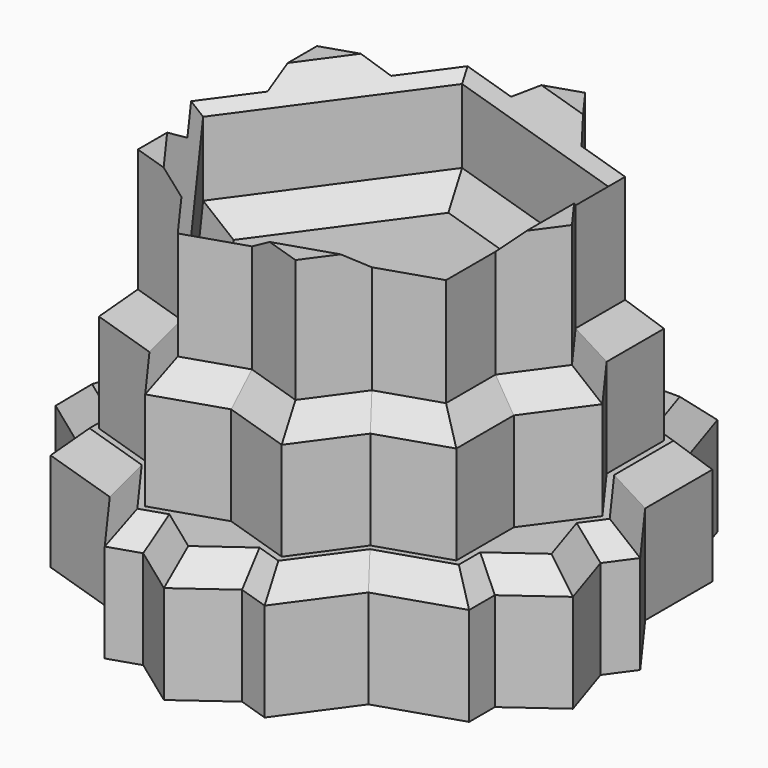
from build123d import *

# Parameters (mm, degrees)
F1_DEPTH      = 25.4
F2_SIZE       = 5.08
F4_DEPTH      = 25.4
F5_SIZE       = 5.08
F7_DEPTH      = 25.4
F8_SIZE       = 5.08
F9_T4_DEPTH   = 69.3683527658
F9_T10_DEPTH  = 69.3683527658
F9_T16_DEPTH  = 69.3683527658
F9_T22_DEPTH  = 69.3683527658
F9_T28_DEPTH  = 69.3683527658
F9_T35_DEPTH  = 69.3683527658
F9_T41_DEPTH  = 69.3683527658
F9_T50_DEPTH  = 69.3683527658
F9_T56_DEPTH  = 69.3683527658
F9_T65_DEPTH  = 69.3683527658
F9_T71_DEPTH  = 69.3683527658
F9_T80_DEPTH  = 69.3683527658
F9_T86_DEPTH  = 69.3683527658
F9_T95_DEPTH  = 69.3683527658
F9_T101_DEPTH = 69.3683527658


# Not quite as in the source:
# - a fillet or chamfer that OpenCascade refuses, or shapes differently, is made with other operations: its cross-section is extruded or revolved along the edge and cut away or added


with BuildPart() as f1:
    # F0 (on Top) → F1 (new body)
    with BuildSketch(Plane.XY):
        Polygon((43.1581027806, 14.0229176455), (43.1581027806, 31.3561970981), (36.8614204445, 33.40211321), align=None)
        Polygon((49.4547851167, -5.3562779191), (43.1581027806, 14.0229176455), (43.1581027806, -14.0229176455), align=None)
        Polygon((43.1581027806, -14.0229176455), (43.1581027806, 14.0229176455), (26.6731744084, 36.7124750172), (0, 45.3791147436), (-26.6731744084, 36.7124750172), (-43.1581027806, 14.0229176455), (-43.1581027806, -14.0229176455), (-26.6731744084, -36.7124750172), (0, -45.3791147436), (26.6731744084, -36.7124750172), align=None)
        Polygon((26.6731744084, 36.7124750172), (43.1581027806, 14.0229176455), (36.8614204445, 33.40211321), align=None)
        Polygon((53.3463488167, 0), (43.1581027806, 14.0229176455), (49.4547851167, -5.3562779191), align=None)
        Polygon((26.6731744084, 36.7124750172), (36.8614204445, 33.40211321), (32.9698567444, 45.3791147436), (20.3764920723, 45.3791147436), align=None)
        Polygon((49.4547851167, -5.3562779191), (43.1581027806, -14.0229176455), (43.1581027806, -24.7354734837), (53.3463488167, -17.3332794527), align=None)
        Polygon((43.1581027806, -24.7354734837), (43.1581027806, -14.0229176455), (26.6731744084, -36.7124750172), align=None)
        Polygon((0, 45.3791147436), (26.6731744084, 36.7124750172), (20.3764920723, 45.3791147436), align=None)
        Polygon((43.1581027806, -31.3561970981), (43.1581027806, -24.7354734837), (26.6731744084, -36.7124750172), align=None)
        Polygon((10.1882460361, -48.6894765508), (26.6731744084, -36.7124750172), (0, -45.3791147436), align=None)
        Polygon((16.4849283722, -50.7353926627), (26.6731744084, -36.7124750172), (10.1882460361, -48.6894765508), align=None)
        Polygon((-20.3764920723, 45.3791147436), (0, 45.3791147436), (-16.4849283722, 50.7353926627), align=None)
        Polygon((-26.6731744084, 36.7124750172), (0, 45.3791147436), (-20.3764920723, 45.3791147436), align=None)
        Polygon((16.4849283722, 50.7353926627), (0, 45.3791147436), (20.3764920723, 45.3791147436), align=None)
        Polygon((10.1882460361, -48.6894765508), (0, -45.3791147436), (-10.1882460361, -48.6894765508), (0, -56.0916705818), align=None)
        Polygon((-10.1882460361, -48.6894765508), (0, -45.3791147436), (-26.6731744084, -36.7124750172), align=None)
        Polygon((-36.8614204445, 33.40211321), (-26.6731744084, 36.7124750172), (-20.3764920723, 45.3791147436), (-32.9698567444, 45.3791147436), align=None)
        Polygon((-43.1581027806, 14.0229176455), (-26.6731744084, 36.7124750172), (-36.8614204445, 33.40211321), align=None)
        Polygon((-16.4849283722, -50.7353926627), (-10.1882460361, -48.6894765508), (-26.6731744084, -36.7124750172), align=None)
        Polygon((-43.1581027806, -24.7354734837), (-26.6731744084, -36.7124750172), (-43.1581027806, -14.0229176455), align=None)
        Polygon((-43.1581027806, -31.3561970981), (-26.6731744084, -36.7124750172), (-43.1581027806, -24.7354734837), align=None)
        Polygon((-49.4547851167, -5.3562779191), (-43.1581027806, 14.0229176455), (-53.3463488167, 0), align=None)
        Polygon((-43.1581027806, -14.0229176455), (-43.1581027806, 14.0229176455), (-49.4547851167, -5.3562779191), align=None)
        Polygon((-43.1581027806, 31.3561970981), (-43.1581027806, 14.0229176455), (-36.8614204445, 33.40211321), align=None)
        Polygon((-43.1581027806, -24.7354734837), (-43.1581027806, -14.0229176455), (-49.4547851167, -5.3562779191), (-53.3463488167, -17.3332794527), align=None)
    extrude(amount=F1_DEPTH)

    # F2
    f2_edges = [f1.edges().sort_by_distance(p)[0] for p in [
        (43.158103, 22.689557, 25.4),
        (40.009762, 32.379155, 25.4),
        (34.915639, 39.390614, 25.4),
        (26.673174, 45.379115, 25.4),
        (18.43071, 48.057254, 25.4),
        (8.242464, 48.057254, 25.4),
        (-8.242464, 48.057254, 25.4),
        (-18.43071, 48.057254, 25.4),
        (-26.673174, 45.379115, 25.4),
        (-34.915639, 39.390614, 25.4),
        (-40.009762, 32.379155, 25.4),
        (-43.158103, 22.689557, 25.4),
        (-48.252226, 7.011459, 25.4),
        (-51.400567, -2.678139, 25.4),
        (-51.400567, -11.344779, 25.4),
        (-48.252226, -21.034376, 25.4),
        (-43.158103, -28.045835, 25.4),
        (-34.915639, -34.034336, 25.4),
        (-21.579051, -43.723934, 25.4),
        (-13.336587, -49.712435, 25.4),
        (-5.094123, -52.390574, 25.4),
        (5.094123, -52.390574, 25.4),
        (13.336587, -49.712435, 25.4),
        (21.579051, -43.723934, 25.4),
        (34.915639, -34.034336, 25.4),
        (43.158103, -28.045835, 25.4),
        (48.252226, -21.034376, 25.4),
        (51.400567, -11.344779, 25.4),
        (51.400567, -2.678139, 25.4),
        (48.252226, 7.011459, 25.4),
    ]]
    chamfer(f2_edges, length=F2_SIZE)

    # F3 (on face) → F4 (join)
    with BuildSketch(Plane.XY.offset(25.4)):
        Polygon((36.8518978357, 11.9739074504), (36.8518978357, 26.7744710154), (22.7757254124, 31.3480966833), align=None)
        Polygon((45.5514508248, 0), (36.8518978357, 11.9739074504), (36.8518978357, -11.9739074504), align=None)
        Polygon((36.8518978357, -11.9739074504), (36.8518978357, 11.9739074504), (22.7757254124, 31.3480966833), (0, 38.7483784658), (-22.7757254124, 31.3480966833), (-36.8518978357, 11.9739074504), (-36.8518978357, -11.9739074504), (-22.7757254124, -31.3480966833), (0, -38.7483784658), (22.7757254124, -31.3480966833), align=None)
        Polygon((0, 38.7483784658), (22.7757254124, 31.3480966833), (14.0761724233, 43.3220041337), align=None)
        Polygon((36.8518978357, -26.7744710154), (36.8518978357, -11.9739074504), (22.7757254124, -31.3480966833), align=None)
        Polygon((-22.7757254124, 31.3480966833), (0, 38.7483784658), (-14.0761724233, 43.3220041337), align=None)
        Polygon((14.0761724233, -43.3220041337), (22.7757254124, -31.3480966833), (0, -38.7483784658), align=None)
        Polygon((-36.8518978357, 11.9739074504), (-22.7757254124, 31.3480966833), (-36.8518978357, 26.7744710154), align=None)
        Polygon((-14.0761724233, -43.3220041337), (0, -38.7483784658), (-22.7757254124, -31.3480966833), align=None)
        Polygon((-36.8518978357, -11.9739074504), (-36.8518978357, 11.9739074504), (-45.5514508248, 0), align=None)
        Polygon((-36.8518978357, -26.7744710154), (-22.7757254124, -31.3480966833), (-36.8518978357, -11.9739074504), align=None)
    extrude(amount=F4_DEPTH)

    # F5
    f5_edges = [f1.edges().sort_by_distance(p)[0] for p in [
        (36.851898, 19.374189, 50.8),
        (29.813812, 29.061284, 50.8),
        (18.425949, 37.33505, 50.8),
        (7.038086, 41.035191, 50.8),
        (-7.038086, 41.035191, 50.8),
        (-18.425949, 37.33505, 50.8),
        (-29.813812, 29.061284, 50.8),
        (-36.851898, 19.374189, 50.8),
        (-41.201674, 5.986954, 50.8),
        (-41.201674, -5.986954, 50.8),
        (-36.851898, -19.374189, 50.8),
        (-29.813812, -29.061284, 50.8),
        (-18.425949, -37.33505, 50.8),
        (-7.038086, -41.035191, 50.8),
        (7.038086, -41.035191, 50.8),
        (18.425949, -37.33505, 50.8),
        (29.813812, -29.061284, 50.8),
        (36.851898, -19.374189, 50.8),
        (41.201674, -5.986954, 50.8),
        (41.201674, 5.986954, 50.8),
    ]]
    chamfer(f5_edges, length=F5_SIZE)

    # F6 (on face) → F7 (join)
    with BuildSketch(Plane.XY.offset(50.8)):
        Polygon((39.2722254991, 0), (31.7718978357, 10.3233153935), (31.7718978357, 23.0836349731), (19.6361127496, 27.0267905768), (12.1357850862, 37.3501059704), (0, 33.4069503666), (-12.1357850862, 37.3501059704), (-19.6361127496, 27.0267905768), (-31.7718978357, 23.0836349731), (-31.7718978357, 10.3233153935), (-39.2722254991, 0), (-31.7718978357, -10.3233153935), (-31.7718978357, -23.0836349731), (-19.6361127496, -27.0267905768), (-12.1357850862, -37.3501059704), (0, -33.4069503666), (12.1357850862, -37.3501059704), (19.6361127496, -27.0267905768), (31.7718978357, -23.0836349731), (31.7718978357, -10.3233153935), align=None)
        Polygon((-11.3663207357, 34.9819382066), (29.7574140131, 21.620026804), (29.7574140131, -21.620026804), (-11.3663207357, -34.9819382066), (-36.7821865549, 0), align=None, mode=Mode.SUBTRACT)
    extrude(amount=F7_DEPTH)

    # F8
    f8_edges = [f1.edges().sort_by_distance(p)[0] for p in [
        (9.195547, 28.300983, 50.8),
        (29.757414, 0, 50.8),
        (9.195547, -28.300983, 50.8),
        (-24.074254, -17.490969, 50.8),
        (-24.074254, 17.490969, 50.8),
    ]]
    chamfer(f8_edges, length=F8_SIZE)

    # F9: chamfer of 5.08 on 5 edges, made by hand


with BuildPart() as f9_tool2:
    # F9_s3 → F9_t4 (new body)
    with BuildSketch(Plane(origin=(-20.3868473658, -28.0600881296, 0), x_dir=(0, 0, 1), z_dir=(0.5877852523, 0.8090169944, 0))):
        Polygon((71.12, -29.7574140131), (76.2, -34.8374140131), (76.2, -29.7574140131), align=None)
    extrude(amount=F9_T4_DEPTH)

    split(bisect_by=Plane(origin=(9.1955466387, 28.3009825053, 0), x_dir=(0, 0, 1), z_dir=(-0.3090169944, -0.9510565163, 0)), keep=Keep.TOP)

    split(bisect_by=Plane(origin=(-24.0742536453, -17.4909691033, 0), x_dir=(0, 0, 1), z_dir=(0.8090169944, 0.5877852523, 0)), keep=Keep.TOP)


with BuildPart() as f1_1:
    add(f1.part)

    # F9_t1: cut F9_tool2
    add(f9_tool2.part, mode=Mode.SUBTRACT)


with BuildPart() as f9_tool8:
    # F9_s9 → F9_t10 (new body)
    with BuildSketch(Plane(origin=(-32.9866119613, 10.7179999382, 0), x_dir=(0, 0, 1), z_dir=(0.9510565163, -0.3090169944, 0))):
        Polygon((71.12, -29.7574140131), (76.2, -34.8374140131), (76.2, -29.7574140131), align=None)
    extrude(amount=F9_T10_DEPTH)

    split(bisect_by=Plane(origin=(-24.0742536453, 17.4909691033, 0), x_dir=(0, 0, 1), z_dir=(0.8090169944, -0.5877852523, 0)), keep=Keep.TOP)

    split(bisect_by=Plane.YZ.offset(29.7574140131), keep=Keep.BOTTOM)


with BuildPart() as f1_2:
    add(f1_1.part)

    # F9_t7: cut F9_tool8
    add(f9_tool8.part, mode=Mode.SUBTRACT)


with BuildPart() as f9_tool14:
    # F9_s15 → F9_t16 (new body)
    with BuildSketch(Plane.XZ.offset(-34.6841763829)):
        Polygon((34.8374140131, 76.2), (29.7574140131, 71.12), (29.7574140131, 76.2), align=None)
    extrude(amount=F9_T16_DEPTH)

    split(bisect_by=Plane(origin=(9.1955466387, 28.3009825053, 0), x_dir=(0, 0, 1), z_dir=(-0.3090169944, -0.9510565163, 0)), keep=Keep.TOP)

    split(bisect_by=Plane(origin=(9.1955466387, -28.3009825053, 0), x_dir=(0, 0, 1), z_dir=(-0.3090169944, 0.9510565163, 0)), keep=Keep.TOP)


with BuildPart() as f1_3:
    add(f1_2.part)

    # F9_t13: cut F9_tool14
    add(f9_tool14.part, mode=Mode.SUBTRACT)


with BuildPart() as f9_tool20:
    # F9_s21 → F9_t22 (new body)
    with BuildSketch(Plane(origin=(32.9866119613, 10.7179999382, 0), x_dir=(0, 0, 1), z_dir=(-0.9510565163, -0.3090169944, 0))):
        Polygon((76.2, -34.8374140131), (71.12, -29.7574140131), (76.2, -29.7574140131), align=None)
    extrude(amount=F9_T22_DEPTH)

    split(bisect_by=Plane.YZ.offset(29.7574140131), keep=Keep.BOTTOM)

    split(bisect_by=Plane(origin=(-24.0742536453, -17.4909691033, 0), x_dir=(0, 0, 1), z_dir=(0.8090169944, 0.5877852523, 0)), keep=Keep.TOP)


with BuildPart() as f1_4:
    add(f1_3.part)

    # F9_t19: cut F9_tool20
    add(f9_tool20.part, mode=Mode.SUBTRACT)


with BuildPart() as f9_tool26:
    # F9_s27 → F9_t28 (new body)
    with BuildSketch(Plane(origin=(20.3868473658, -28.0600881296, 0), x_dir=(0, 0, 1), z_dir=(-0.5877852523, 0.8090169944, 0))):
        Polygon((76.2, -34.8374140131), (71.12, -29.7574140131), (76.2, -29.7574140131), align=None)
    extrude(amount=F9_T28_DEPTH)

    split(bisect_by=Plane(origin=(-24.0742536453, 17.4909691033, 0), x_dir=(0, 0, 1), z_dir=(0.8090169944, -0.5877852523, 0)), keep=Keep.TOP)

    split(bisect_by=Plane(origin=(9.1955466387, -28.3009825053, 0), x_dir=(0, 0, 1), z_dir=(-0.3090169944, 0.9510565163, 0)), keep=Keep.TOP)


with BuildPart() as f1_5:
    add(f1_4.part)

    # F9_t25: cut F9_tool26
    add(f9_tool26.part, mode=Mode.SUBTRACT)


with BuildPart() as f9_tool33:
    # F9_s34 → F9_t35 (new body)
    with BuildSketch(Plane(origin=(-20.3868473658, -28.0600881296, 0), x_dir=(0, 0, 1), z_dir=(0.5877852523, 0.8090169944, 0))):
        Polygon((71.12, -29.7574140131), (76.2, -34.8374140131), (76.2, -29.7574140131), align=None)
    extrude(amount=F9_T35_DEPTH)

    split(bisect_by=Plane(origin=(-24.0742536453, -17.4909691033, 0), x_dir=(0, 0, 1), z_dir=(-0.8090169944, -0.5877852523, 0)), keep=Keep.TOP)

    split(bisect_by=Plane(origin=(-25.7040052927, 18.6750529852, 0), x_dir=(0, 0, 1), z_dir=(0.8090169944, -0.5877852523, 0)), keep=Keep.TOP)

    split(bisect_by=Plane(origin=(-25.7040052927, -18.6750529852, 0), x_dir=(0, 0, 1), z_dir=(0.8090169944, 0.5877852523, 0)), keep=Keep.TOP)


with BuildPart() as f9_tool39:
    # F9_s40 → F9_t41 (new body)
    with BuildSketch(Plane(origin=(20.3868473658, -28.0600881296, 0), x_dir=(0, 0, 1), z_dir=(-0.5877852523, 0.8090169944, 0))):
        Polygon((76.2, -34.8374140131), (71.12, -29.7574140131), (76.2, -29.7574140131), align=None)
    extrude(amount=F9_T41_DEPTH)

    split(bisect_by=Plane(origin=(-24.0742536453, 17.4909691033, 0), x_dir=(0, 0, 1), z_dir=(-0.8090169944, 0.5877852523, 0)), keep=Keep.TOP)

    split(bisect_by=Plane(origin=(-25.7040052927, 18.6750529852, 0), x_dir=(0, 0, 1), z_dir=(0.8090169944, -0.5877852523, 0)), keep=Keep.TOP)

    split(bisect_by=Plane(origin=(-25.7040052927, -18.6750529852, 0), x_dir=(0, 0, 1), z_dir=(0.8090169944, 0.5877852523, 0)), keep=Keep.TOP)


with BuildPart() as f9_tool33_1:
    add(f9_tool33.part)

    # F9_t45: intersect F9_tool39
    add(f9_tool39.part, mode=Mode.INTERSECT)


with BuildPart() as f1_6:
    add(f1_5.part)

    # F9_t31: cut F9_tool33
    add(f9_tool33_1.part, mode=Mode.SUBTRACT)


with BuildPart() as f9_tool48:
    # F9_s49 → F9_t50 (new body)
    with BuildSketch(Plane(origin=(-32.9866119613, 10.7179999382, 0), x_dir=(0, 0, 1), z_dir=(0.9510565163, -0.3090169944, 0))):
        Polygon((71.12, -29.7574140131), (76.2, -34.8374140131), (76.2, -29.7574140131), align=None)
    extrude(amount=F9_T50_DEPTH)

    split(bisect_by=Plane(origin=(-24.0742536453, 17.4909691033, 0), x_dir=(0, 0, 1), z_dir=(-0.8090169944, 0.5877852523, 0)), keep=Keep.TOP)

    split(bisect_by=Plane(origin=(9.8180563748, 30.2168704717, 0), x_dir=(0, 0, 1), z_dir=(-0.3090169944, -0.9510565163, 0)), keep=Keep.TOP)

    split(bisect_by=Plane(origin=(-25.7040052927, 18.6750529852, 0), x_dir=(0, 0, 1), z_dir=(0.8090169944, -0.5877852523, 0)), keep=Keep.TOP)


with BuildPart() as f9_tool54:
    # F9_s55 → F9_t56 (new body)
    with BuildSketch(Plane(origin=(-20.3868473658, -28.0600881296, 0), x_dir=(0, 0, 1), z_dir=(0.5877852523, 0.8090169944, 0))):
        Polygon((71.12, -29.7574140131), (76.2, -34.8374140131), (76.2, -29.7574140131), align=None)
    extrude(amount=F9_T56_DEPTH)

    split(bisect_by=Plane(origin=(9.1955466387, 28.3009825053, 0), x_dir=(0, 0, 1), z_dir=(0.3090169944, 0.9510565163, 0)), keep=Keep.TOP)

    split(bisect_by=Plane(origin=(9.8180563748, 30.2168704717, 0), x_dir=(0, 0, 1), z_dir=(-0.3090169944, -0.9510565163, 0)), keep=Keep.TOP)

    split(bisect_by=Plane(origin=(-25.7040052927, 18.6750529852, 0), x_dir=(0, 0, 1), z_dir=(0.8090169944, -0.5877852523, 0)), keep=Keep.TOP)


with BuildPart() as f9_tool48_1:
    add(f9_tool48.part)

    # F9_t60: intersect F9_tool54
    add(f9_tool54.part, mode=Mode.INTERSECT)


with BuildPart() as f1_7:
    add(f1_6.part)

    # F9_t46: cut F9_tool48
    add(f9_tool48_1.part, mode=Mode.SUBTRACT)


with BuildPart() as f9_tool63:
    # F9_s64 → F9_t65 (new body)
    with BuildSketch(Plane(origin=(-32.9866119613, 10.7179999382, 0), x_dir=(0, 0, 1), z_dir=(0.9510565163, -0.3090169944, 0))):
        Polygon((71.12, -29.7574140131), (76.2, -34.8374140131), (76.2, -29.7574140131), align=None)
    extrude(amount=F9_T65_DEPTH)

    split(bisect_by=Plane.YZ.offset(29.7574140131), keep=Keep.TOP)

    split(bisect_by=Plane.YZ.offset(31.7718978357), keep=Keep.BOTTOM)

    split(bisect_by=Plane(origin=(9.8180563748, 30.2168704717, 0), x_dir=(0, 0, 1), z_dir=(-0.3090169944, -0.9510565163, 0)), keep=Keep.TOP)


with BuildPart() as f9_tool69:
    # F9_s70 → F9_t71 (new body)
    with BuildSketch(Plane.XZ.offset(-34.6841763829)):
        Polygon((34.8374140131, 76.2), (29.7574140131, 71.12), (29.7574140131, 76.2), align=None)
    extrude(amount=F9_T71_DEPTH)

    split(bisect_by=Plane(origin=(9.1955466387, 28.3009825053, 0), x_dir=(0, 0, 1), z_dir=(0.3090169944, 0.9510565163, 0)), keep=Keep.TOP)

    split(bisect_by=Plane.YZ.offset(31.7718978357), keep=Keep.BOTTOM)

    split(bisect_by=Plane(origin=(9.8180563748, 30.2168704717, 0), x_dir=(0, 0, 1), z_dir=(-0.3090169944, -0.9510565163, 0)), keep=Keep.TOP)


with BuildPart() as f9_tool63_1:
    add(f9_tool63.part)

    # F9_t75: intersect F9_tool69
    add(f9_tool69.part, mode=Mode.INTERSECT)


with BuildPart() as f1_8:
    add(f1_7.part)

    # F9_t61: cut F9_tool63
    add(f9_tool63_1.part, mode=Mode.SUBTRACT)


with BuildPart() as f9_tool78:
    # F9_s79 → F9_t80 (new body)
    with BuildSketch(Plane.XZ.offset(-34.6841763829)):
        Polygon((34.8374140131, 76.2), (29.7574140131, 71.12), (29.7574140131, 76.2), align=None)
    extrude(amount=F9_T80_DEPTH)

    split(bisect_by=Plane(origin=(9.8180563748, -30.2168704717, 0), x_dir=(0, 0, 1), z_dir=(-0.3090169944, 0.9510565163, 0)), keep=Keep.TOP)

    split(bisect_by=Plane.YZ.offset(31.7718978357), keep=Keep.BOTTOM)

    split(bisect_by=Plane(origin=(9.1955466387, -28.3009825053, 0), x_dir=(0, 0, 1), z_dir=(0.3090169944, -0.9510565163, 0)), keep=Keep.TOP)


with BuildPart() as f9_tool84:
    # F9_s85 → F9_t86 (new body)
    with BuildSketch(Plane(origin=(32.9866119613, 10.7179999382, 0), x_dir=(0, 0, 1), z_dir=(-0.9510565163, -0.3090169944, 0))):
        Polygon((76.2, -34.8374140131), (71.12, -29.7574140131), (76.2, -29.7574140131), align=None)
    extrude(amount=F9_T86_DEPTH)

    split(bisect_by=Plane.YZ.offset(29.7574140131), keep=Keep.TOP)

    split(bisect_by=Plane(origin=(9.8180563748, -30.2168704717, 0), x_dir=(0, 0, 1), z_dir=(-0.3090169944, 0.9510565163, 0)), keep=Keep.TOP)

    split(bisect_by=Plane.YZ.offset(31.7718978357), keep=Keep.BOTTOM)


with BuildPart() as f9_tool78_1:
    add(f9_tool78.part)

    # F9_t90: intersect F9_tool84
    add(f9_tool84.part, mode=Mode.INTERSECT)


with BuildPart() as f1_9:
    add(f1_8.part)

    # F9_t76: cut F9_tool78
    add(f9_tool78_1.part, mode=Mode.SUBTRACT)


with BuildPart() as f9_tool93:
    # F9_s94 → F9_t95 (new body)
    with BuildSketch(Plane(origin=(32.9866119613, 10.7179999382, 0), x_dir=(0, 0, 1), z_dir=(-0.9510565163, -0.3090169944, 0))):
        Polygon((76.2, -34.8374140131), (71.12, -29.7574140131), (76.2, -29.7574140131), align=None)
    extrude(amount=F9_T95_DEPTH)

    split(bisect_by=Plane(origin=(-24.0742536453, -17.4909691033, 0), x_dir=(0, 0, 1), z_dir=(-0.8090169944, -0.5877852523, 0)), keep=Keep.TOP)

    split(bisect_by=Plane(origin=(9.8180563748, -30.2168704717, 0), x_dir=(0, 0, 1), z_dir=(-0.3090169944, 0.9510565163, 0)), keep=Keep.TOP)

    split(bisect_by=Plane(origin=(-25.7040052927, -18.6750529852, 0), x_dir=(0, 0, 1), z_dir=(0.8090169944, 0.5877852523, 0)), keep=Keep.TOP)


with BuildPart() as f9_tool99:
    # F9_s100 → F9_t101 (new body)
    with BuildSketch(Plane(origin=(20.3868473658, -28.0600881296, 0), x_dir=(0, 0, 1), z_dir=(-0.5877852523, 0.8090169944, 0))):
        Polygon((76.2, -34.8374140131), (71.12, -29.7574140131), (76.2, -29.7574140131), align=None)
    extrude(amount=F9_T101_DEPTH)

    split(bisect_by=Plane(origin=(-25.7040052927, -18.6750529852, 0), x_dir=(0, 0, 1), z_dir=(0.8090169944, 0.5877852523, 0)), keep=Keep.TOP)

    split(bisect_by=Plane(origin=(9.8180563748, -30.2168704717, 0), x_dir=(0, 0, 1), z_dir=(-0.3090169944, 0.9510565163, 0)), keep=Keep.TOP)

    split(bisect_by=Plane(origin=(9.1955466387, -28.3009825053, 0), x_dir=(0, 0, 1), z_dir=(0.3090169944, -0.9510565163, 0)), keep=Keep.TOP)


with BuildPart() as f9_tool93_1:
    add(f9_tool93.part)

    # F9_t105: intersect F9_tool99
    add(f9_tool99.part, mode=Mode.INTERSECT)


with BuildPart() as f1_10:
    add(f1_9.part)

    # F9_t91: cut F9_tool93
    add(f9_tool93_1.part, mode=Mode.SUBTRACT)


solid = f1_10.part
